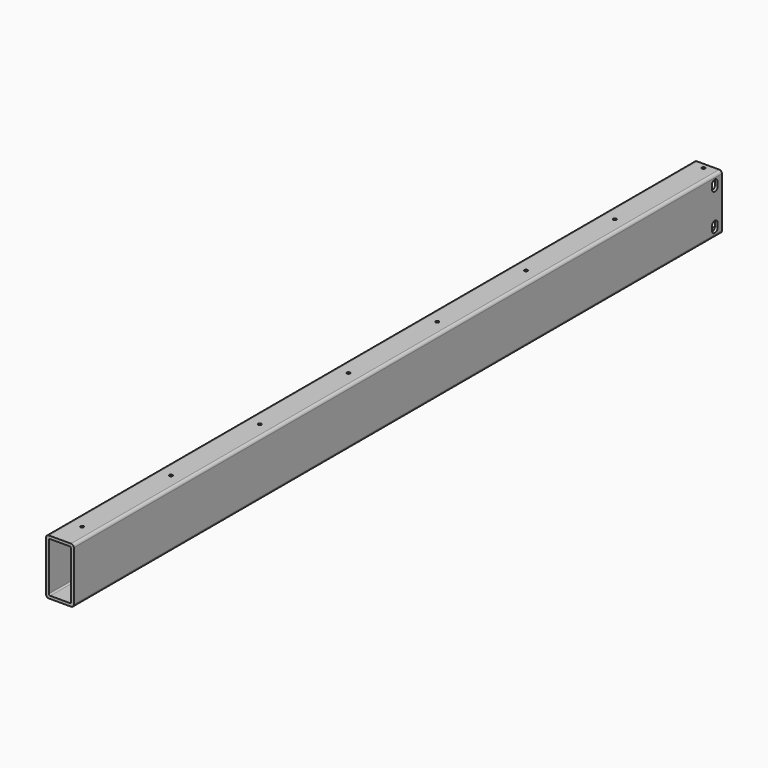
from build123d import *

# Parameters (mm, degrees)
F1_DEPTH = 1460
F3_D     = 5.5
F3_DEPTH = 14.4
F3_TIP   = 1.6523667023
F5_DEPTH = 50.001


# Not quite as in the source:
# - a feature names something its author has since deleted; it is built from what else it names


with BuildPart() as f1:
    # F0 (on Front) → F1 (new body)
    with BuildSketch(Plane.XZ):
        with BuildLine():
            Line((-20, -50), (20, -50))
            ThreePointArc((20, -50), (23.5355339059, -48.5355339059), (25, -45))
            Line((25, -45), (25, 45))
            ThreePointArc((25, 45), (23.5355339059, 48.5355339059), (20, 50))
            Line((20, 50), (-20, 50))
            ThreePointArc((-20, 50), (-23.5355339059, 48.5355339059), (-25, 45))
            Line((-25, 45), (-25, -45))
            ThreePointArc((-25, -45), (-23.5355339059, -48.5355339059), (-20, -50))
        make_face()
        with BuildLine():
            ThreePointArc((-17.5, -45), (-19.267766953, -44.267766953), (-20, -42.5))
            Line((-20, -42.5), (-20, 42.5))
            ThreePointArc((-20, 42.5), (-19.267766953, 44.267766953), (-17.5, 45))
            Line((-17.5, 45), (17.5, 45))
            ThreePointArc((17.5, 45), (19.267766953, 44.267766953), (20, 42.5))
            Line((20, 42.5), (20, -42.5))
            ThreePointArc((20, -42.5), (19.267766953, -44.267766953), (17.5, -45))
            Line((17.5, -45), (-17.5, -45))
        make_face(mode=Mode.SUBTRACT)
    extrude(amount=-F1_DEPTH)

    # F3
    with Locations(Plane.XY.offset(50)):
        with Locations((0, 50), (0, 250), (0, 450), (0, 650), (0, 850), (0, 1050), (0, 1250), (0, 1450)):
            Hole(F3_D / 2, depth=F3_DEPTH)
            with Locations((0, 0, -(F3_DEPTH + F3_TIP / 2))):  # 118° drill point
                Cone(0, F3_D / 2, F3_TIP, mode=Mode.SUBTRACT)

    # F4 (on face) → F5 (cut, through all)
    with BuildSketch(Plane.YZ.offset(25)):
        with BuildLine():
            Line((1450.4894832185, 29.8696045958), (1450.4894832185, 35.6303954042))
            ThreePointArc((1450.4894832185, 35.6303954042), (1444.1498086534, 42.4982734143), (1437.5003786468, 35.9298411402))
            Line((1437.5003786468, 35.9298411402), (1437.5003786468, 29.5701588598))
            ThreePointArc((1437.5003786468, 29.5701588598), (1444.1498086534, 23.0017265857), (1450.4894832185, 29.8696045958))
        make_face()
        with BuildLine():
            Line((1437.5008297564, -29.6038563662), (1437.5000000547, -35.999156715))
            ThreePointArc((1437.5000000547, -35.999156715), (1444.0002415297, -42.4999999955), (1450.4999998647, -35.9986736556))
            Line((1450.4999998647, -35.9986736556), (1450.4987003133, -29.6299778371))
            ThreePointArc((1450.4987003133, -29.6299778371), (1444.0130628488, -23.000013126), (1437.5008297564, -29.6038563662))
        make_face()
    extrude(amount=-F5_DEPTH, mode=Mode.SUBTRACT)


solid = f1.part
